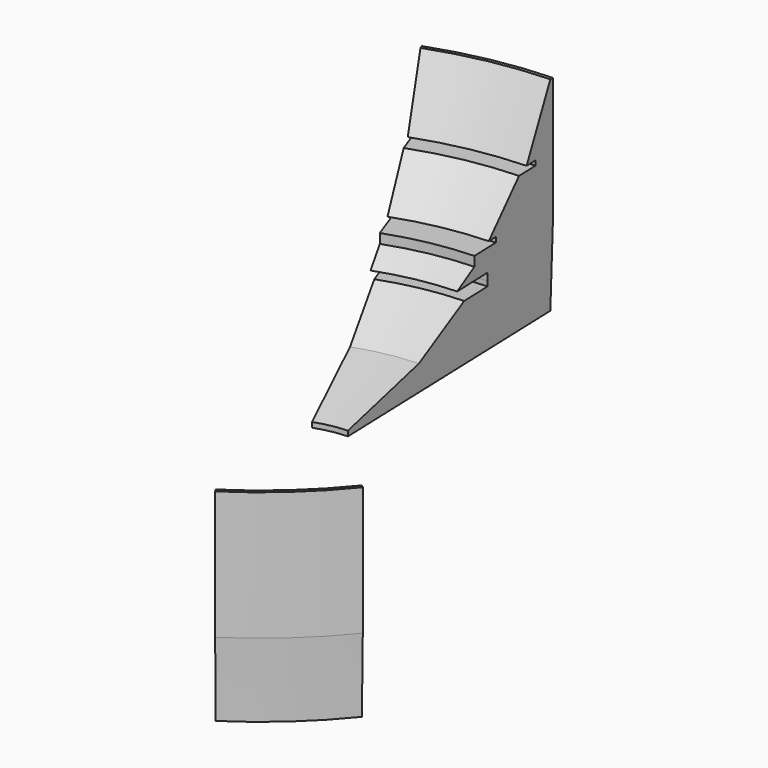
from build123d import *

# Parameters (mm, degrees)
F3_ANGLE_START = 250
F3_ANGLE       = 17.9876048978


with BuildPart() as f3:
    # F0 (on Front) → F3 (revolve)
    with BuildSketch(Plane.XZ, mode=Mode.PRIVATE) as f3_sk:
        Polygon((120, 10), (120, 0), (355.2403748035, 0), (642.4294114113, 0), (648.8609313965, 148.714363575), (648.8609313965, 402.0894765854), (642.4294114113, 402.0894765854), (581.1189413071, 277.4473130703), (604.0261387825, 277.4473130703), (604.0261387825, 268.1565284729), (575.0552415848, 268.1565284729), (561.5838170052, 268.1565284729), (483.4298193455, 187.307536602), (501.6208291054, 187.307536602), (501.6208291054, 177.2014200687), (446.3740289211, 177.2014200687), (446.3740289211, 158.3366543055), (401.9070863724, 134.0060383081), (420, 134.0060383081), (480.7348549366, 134.0060383081), (480.3846478462, 119.7138205171), (480.3846478462, 110), (420, 110), (303.1612038612, 50.1583777368), align=None)
    revolve(f3_sk.sketch.rotate(Axis((-80, 0, 35.9871760011), (0, 0, -1)), F3_ANGLE_START), axis=Axis((-80, 0, 35.9871760011), (0, 0, -1)), revolution_arc=F3_ANGLE)


with BuildPart() as f5_1:
    # F5: instance of F3
    add(f3.part.mirror(Plane(origin=(0, 0, 0), x_dir=(0.894427191, 0.4472135955, 0), z_dir=(0.4472135955, -0.894427191, 0))))


solid = Compound([f3.part, f5_1.part])
